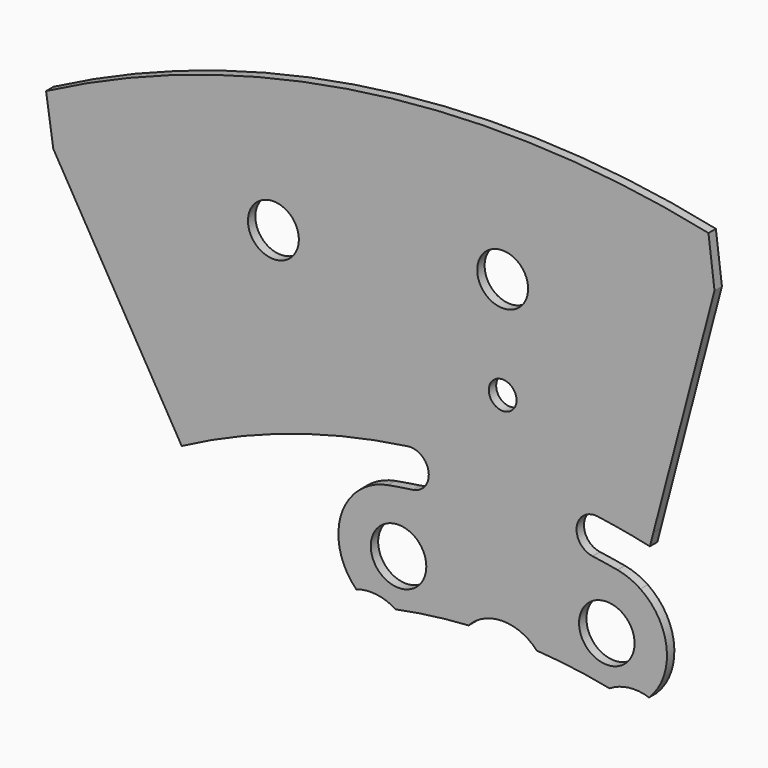
from build123d import *

# Parameters (mm, degrees)
F0_R     = 3
F0_R_2   = 2.75
F0_R_3   = 1.5
F1_DEPTH = 1


# Not quite as in the source:
# - ends of sketch curves that miss each other by under 0.0002 mm in the source are joined


with BuildPart() as f1:
    # F0 (on Front) → F1 (new body)
    with BuildSketch(Plane.XZ):
        with BuildLine():
            ThreePointArc((10.2610980266, 73.2851271902), (13.0931802752, 72.8324696154), (15.9055950445, 72.2704092024))
            Line((15.9055950445, 72.2704092024), (16.286797, 73.722386))
            Line((16.286797, 73.722386), (22.888167, 98.86666))
            Line((22.888167, 98.86666), (22.234036, 104.134663))
            ThreePointArc((22.234036, 104.134663), (-14.4021915305, 105.5033516635), (-49.3311389264, 94.3653488593))
            Line((-49.3311389264, 94.3653488593), (-48.548236, 89.117403))
            Line((-48.548236, 89.117403), (-35.435226, 66.667794))
            Line((-35.435226, 66.667794), (-34.67805, 65.371499))
            ThreePointArc((-34.67805, 65.371499), (-22.8153047874, 70.3950414977), (-10.2610980266, 73.2851271902))
            ThreePointArc((-10.2610980266, 73.2851271902), (-8.0030918925, 71.581775015), (-9.706443985, 69.3237688925))
            ThreePointArc((-9.706443985, 69.3237688925), (-11.056110798, 69.1213600418), (-12.4015749915, 68.8926769529))
            ThreePointArc((-12.4015749915, 68.8926769529), (-13.6918696678, 68.5193918089), (-14.8778891297, 67.8888681928))
            ThreePointArc((-14.8778891297, 67.8888681928), (-17.7216913701, 63.1014792158), (-15.8160679868, 57.8693760134))
            ThreePointArc((-15.8160679868, 57.8693760134), (-13.6269577418, 58.088804993), (-11.5555822107, 57.3473496681))
            ThreePointArc((-11.5555822107, 57.3473496681), (-7.6357821132, 57.9995244077), (-3.6807509947, 58.3840909162))
            ThreePointArc((-3.6807509947, 58.3840909162), (0, 60), (3.6807510132, 58.3840910122))
            ThreePointArc((3.6807510132, 58.3840910122), (7.6357821132, 57.9995244077), (11.5555819538, 57.3473497706))
            ThreePointArc((11.5555819538, 57.3473497706), (13.6269577418, 58.088804993), (15.8160679296, 57.8693757888))
            ThreePointArc((15.8160679296, 57.8693757888), (17.7216913701, 63.1014792158), (14.8778891297, 67.8888681928))
            ThreePointArc((14.8778891297, 67.8888681928), (13.6918696678, 68.5193918089), (12.4015750198, 68.8926771098))
            ThreePointArc((12.4015750198, 68.8926771098), (11.056110798, 69.1213600418), (9.7064439965, 69.3237689753))
            ThreePointArc((9.7064439965, 69.3237689753), (8.0030918925, 71.581775015), (10.2610980266, 73.2851271902))
        make_face()
        with Locations((-11.25, 62.4955)):
            Circle(F0_R, mode=Mode.SUBTRACT)
        with Locations((-24.770679, 89.121622)):
            Circle(F0_R_2, mode=Mode.SUBTRACT)
        with Locations((0, 81.481831)):
            Circle(F0_R_3, mode=Mode.SUBTRACT)
        with Locations((0, 92.5)):
            Circle(F0_R_2, mode=Mode.SUBTRACT)
        with Locations((11.25, 62.4955)):
            Circle(F0_R, mode=Mode.SUBTRACT)
    extrude(amount=F1_DEPTH)


solid = f1.part
